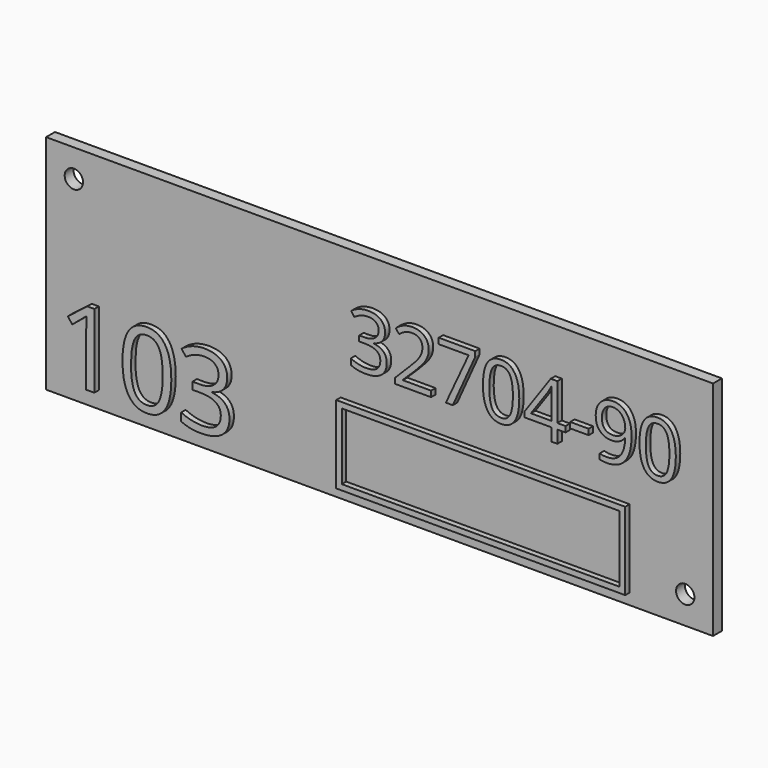
from build123d import *

# Parameters (mm, degrees)
F0_W         = 120
F0_H         = 40
F1_DEPTH     = 2
F3_D         = 3.3
F4_TEXT_SIZE = 13.8283697648
F5_DEPTH     = 1
F6_TEXT_SIZE = 18.5894526641
F7_DEPTH     = 1
F8_W         = 52
F8_H         = 14
F8_W_2       = 49.99999962
F8_H_2       = 11.99999962
F9_DEPTH     = 1


# Not quite as in the source:
# - Text() gives the source's letters only with a copy of the font that has no kerning and outlines rounded to 1/6400 em; it was checked with that copy


with BuildPart() as f1:
    # F0 (on Front) → F1 (new body)
    with BuildSketch(Plane.XZ):
        Rectangle(F0_W, F0_H)
    extrude(amount=F1_DEPTH)

    # F3 (through all)
    with Locations(Plane.XZ.offset(2)):
        with Locations((-55, 15), (55, -15)):
            Hole(F3_D / 2)

    # F4 (on face) → F5 (join)
    with BuildSketch(Plane.XZ.offset(2)):
        with Locations((-5, 2)):
            Text('32704-90', F4_TEXT_SIZE, font='Open Sans', text_align=(TextAlign.LEFT, TextAlign.BOTTOM))
    extrude(amount=F5_DEPTH)

    # F6 (on face) → F7 (join)
    with BuildSketch(Plane.XZ.offset(2)):
        with Locations((-57, -17)):
            Text('103', F6_TEXT_SIZE, font='Open Sans', text_align=(TextAlign.LEFT, TextAlign.BOTTOM))
    extrude(amount=F7_DEPTH)

    # F8 (on face) → F9 (join)
    with BuildSketch(Plane.XZ.offset(2)):
        with Locations((19, -11)):
            Rectangle(F8_W, F8_H)
        with Locations((19, -11)):
            Rectangle(F8_W_2, F8_H_2, mode=Mode.SUBTRACT)
    extrude(amount=F9_DEPTH)


solid = f1.part
